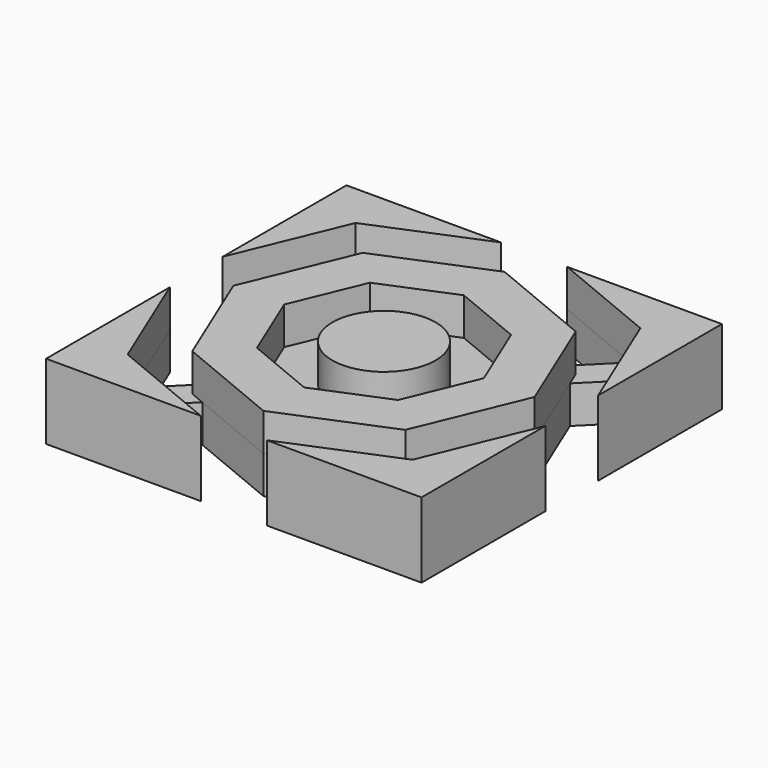
from build123d import *

# Parameters (mm, degrees)
F0_W            = 25.4
F0_H            = 25.4
F1_DEPTH        = 1.27
F3_DEPTH        = 2.54
F2_R            = 3.4925
F4_DEPTH        = 2.54
F5_DEPTH        = 2.54
F5_COPIES_COUNT = 4
F7_DEPTH        = 2.541
F7_COPIES_COUNT = 4


# Not quite as in the source:
# - a pattern or mirror of a feature is missing from the dataset's text; its kind, count and spacing are read off the source's solid


with BuildPart() as f1:
    # F0 (on Top) → F1 (new body, symmetric)
    with BuildSketch(Plane.XY):
        Rectangle(F0_W, F0_H)
    extrude(amount=F1_DEPTH, both=True)

    # F2 (on face) → F3 (join)
    with BuildSketch(Plane.XY.offset(1.27)):
        Polygon((0, 10.1892549187), (-7.2048912482, 7.2048912482), (-10.1892549187, 0), (-7.2048912482, -7.2048912482), (0, -10.1892549187), (7.2048912482, -7.2048912482), (10.1892549187, 0), (7.2048912482, 7.2048912482), align=None)
        Polygon((-4.7748514527, 4.7748514527), (0, 6.7526596828), (4.7748514527, 4.7748514527), (6.7526596828, 0), (4.7748514527, -4.7748514527), (0, -6.7526596828), (-4.7748514527, -4.7748514527), (-6.7526596828, 0), align=None, mode=Mode.SUBTRACT)
    extrude(amount=F3_DEPTH)

    # F2 (on face) → F4 (join, through all)
    with BuildSketch(Plane.XY.offset(1.27)):
        Circle(F2_R)
    extrude(amount=F4_DEPTH)

    # F2 (on face) → F5 (join, through all)
    with BuildSketch(Plane.XY.offset(1.27)):
        Polygon((-2.2352, 12.7), (-12.7, 12.7), (-12.7, 2.2352), (-9.6349310438, 9.6349310438), align=None)
    f5 = extrude(amount=F5_DEPTH)

    # F5_copies: F5 ×4 about axis
    f5_copies_axis = Axis((0, 0, 0), (0, 0, 1))
    for i in range(1, F5_COPIES_COUNT):
        add(f5.rotate(f5_copies_axis, i * 360 / F5_COPIES_COUNT))

    # F6 (on face) → F7 (cut, through all)
    with BuildSketch(Plane.XY.offset(1.27)):
        Polygon((-8.6189310438, 10.0557720231), (-6.1888912482, 7.6257322276), (0, 10.1892549187), (6.1888912482, 7.6257322276), (8.6189310438, 10.0557720231), (2.2352, 12.7), (-2.2352, 12.7), align=None)
    f7 = extrude(amount=-F7_DEPTH, mode=Mode.SUBTRACT)

    # F7_copies: F7 ×4 about axis
    f7_copies_axis = Axis((0, 0, 0), (0, 0, 1))
    for i in range(1, F7_COPIES_COUNT):
        add(f7.rotate(f7_copies_axis, i * 360 / F7_COPIES_COUNT), mode=Mode.SUBTRACT)


solid = f1.part
